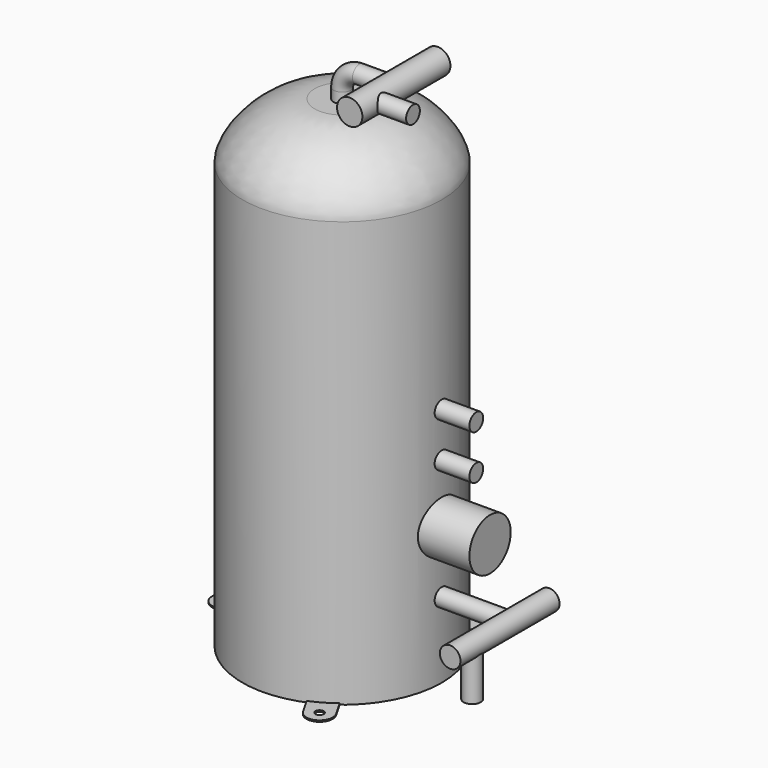
from build123d import *

# Parameters (mm, degrees)
F2_W             = 110
F2_H             = 12.5
F2_W_2           = 80
F2_H_2           = 37.5
F2_W_3           = 60
F8_R             = 12.5
F10_R            = 18.410968248
F11_DEPTH        = 80
F14_R            = 12.5
F15_DEPTH        = 60
F16_R            = 15
F17_DEPTH        = 110
F17_DEPTH_BACK   = 70
F20_R            = 12.5
F21_DEPTH        = 70
F22_R            = 6
F23_DEPTH        = 2
F23_COPIES_COUNT = 3


# Not quite as in the source:
# - a pattern or mirror of a feature is missing from the dataset's text; its kind, count and spacing are read off the source's solid


with BuildPart() as f1:
    # F0 (on Front) → F1 (revolve)
    with BuildSketch(Plane.XZ):
        with BuildLine():
            Line((0, 700), (0, 0))
            Line((0, 0), (145, 0))
            Line((145, 0), (145, 617.9695725441))
            add(Edge.make_bspline(
                [(39.8514680564, 700), (99.0592166781, 698.7452507019), (144.9243873358, 643.1511044502), (145, 617.9695725441)],
                knots=[0, 0, 0, 0, 133.3611817527, 133.3611817527, 133.3611817527, 133.3611817527], degree=3))
            Line((39.8514680564, 700), (0, 700))
        make_face()
    revolve(axis=Axis((0, 0, 350), (0, 0, -1)))

    # F2 (on Front) → F3 (revolve)
    with BuildSketch(Plane.XZ):
        with Locations((190, 116.25)):
            Rectangle(F2_W, F2_H)
    revolve(axis=Axis((190, 0, 110), (1, 0, 0)))

    # F2 (on Front) → F4 (revolve)
    with BuildSketch(Plane.XZ):
        with Locations((175, 218.75)):
            Rectangle(F2_W_2, F2_H_2)
    revolve(axis=Axis((175, 0, 200), (1, 0, 0)))

    # F2 (on Front) → F5 (revolve)
    with BuildSketch(Plane.XZ):
        with Locations((165, 291.25)):
            Rectangle(F2_W_3, F2_H)
    revolve(axis=Axis((165, 0, 285), (1, 0, 0)))

    # F2 (on Front) → F6 (revolve)
    with BuildSketch(Plane.XZ):
        with Locations((165, 356.25)):
            Rectangle(F2_W_3, F2_H)
    revolve(axis=Axis((165, 0, 350), (1, 0, 0)))

    # F9: sweep along a path in F7
    with BuildLine(Plane.XZ) as f9_path:
        Line((0, 700), (0, 715))
        ThreePointArc((0, 715), (7.3223304703, 732.6776695297), (25, 740))
        Line((25, 740), (75, 740))
    # F8 (on face) → F9 (sweep)
    with BuildSketch(Plane.XY.offset(700)):
        Circle(F8_R)
    sweep(path=f9_path.line)

    # F10 (on Front) → F11 (join, symmetric)
    with BuildSketch(Plane.XZ):
        with Locations((75, 740)):
            Circle(F10_R)
    extrude(amount=F11_DEPTH, both=True)

    # F14 (on face) → F15 (join)
    with BuildSketch(Plane(origin=(75, 0, 0), x_dir=(0, -1, 0), z_dir=(-1, 0, 0))):
        with Locations((40, 740)):
            Circle(F14_R)
    extrude(amount=-F15_DEPTH)

    # F16 (on Front) → F17 (join, two sides)
    with BuildSketch(Plane.XZ) as f17_sk:
        with Locations((245, 110)):
            Circle(F16_R)
    extrude(amount=F17_DEPTH)
    extrude(f17_sk.sketch, amount=-F17_DEPTH_BACK)

    # F20 (on face) → F21 (join)
    with BuildSketch(Plane(origin=(0, 0, 110), x_dir=(1, 0, 0), z_dir=(0, 0, -1))):
        with Locations((245, 70)):
            Circle(F20_R)
    extrude(amount=F21_DEPTH)


with BuildPart() as f23:
    # F22 (on face) → F23 (new body)
    with BuildSketch(Plane(origin=(0, 0, 0), x_dir=(1, 0, 0), z_dir=(0, 0, -1))):
        with BuildLine():
            ThreePointArc((101.4544826719, 137.7243186434), (94.5, 163.6788013153), (68.5455173281, 156.7243186434))
            Line((68.5455173281, 156.7243186434), (55.4204086324, 133.9909635275))
            ThreePointArc((55.4204086324, 133.9909635275), (72.5, 125.5736835487), (88.3293739762, 114.9909635275))
            Line((88.3293739762, 114.9909635275), (101.4544826719, 137.7243186434))
        make_face()
        with Locations((85, 147.2243186434)):
            Circle(F22_R, mode=Mode.SUBTRACT)
    extrude(amount=-F23_DEPTH)


with BuildPart() as f23_copies_1:
    # F23_copies: instance of F23
    add(f23.part.rotate(Axis((0, 0, 0), (0, 0, 1)), 1 * 360 / F23_COPIES_COUNT))


with BuildPart() as f23_copies_2:
    # F23_copies: instance of F23
    add(f23.part.rotate(Axis((0, 0, 0), (0, 0, 1)), 2 * 360 / F23_COPIES_COUNT))


solid = Compound([f1.part, f23.part, f23_copies_1.part, f23_copies_2.part])
